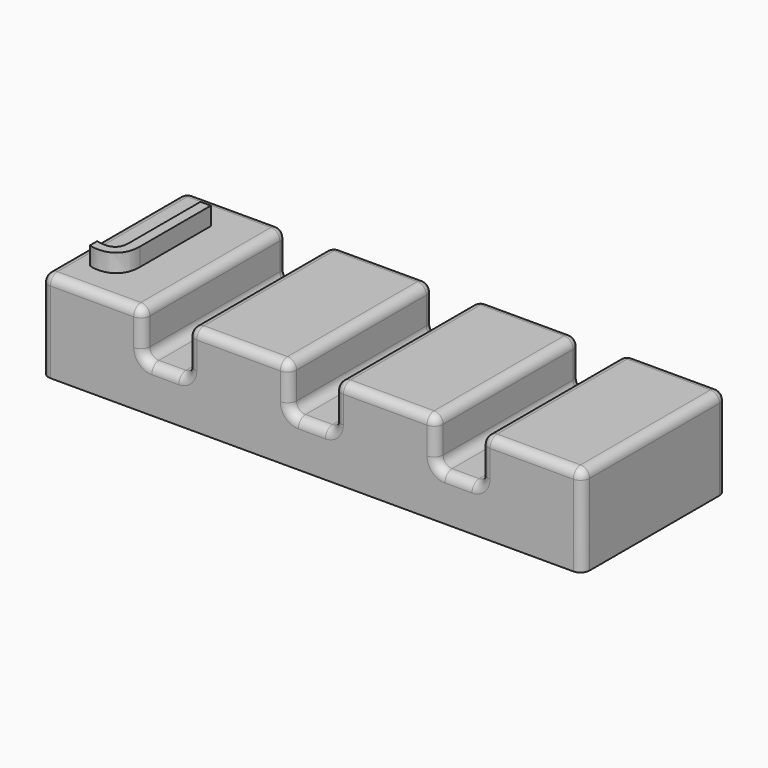
from build123d import *

# Parameters (mm, degrees)
F0_W         = 76.2
F0_H         = 25.4
F1_DEPTH     = 12.7
F2_W         = 6.35
F2_H         = 12.7
F3_DEPTH     = 25.401
F4_R         = 1.27
F5_T         = -2.54
F6_TEXT_SIZE = 17.6218719894
F7_DEPTH     = 2.54


# Not quite as in the source:
# - Text() gives the source's letters only with a copy of the font that has no kerning and outlines rounded to 1/6400 em; it was checked with that copy


with BuildPart() as f1:
    # F0 (on Top) → F1 (new body)
    with BuildSketch(Plane.XY):
        Rectangle(F0_W, F0_H)
    extrude(amount=F1_DEPTH)

    # F2 (on face) → F3 (cut, through all)
    with BuildSketch(Plane.XZ.offset(12.7)):
        with Locations((20.6502, 12.7)):
            Rectangle(F2_W, F2_H)
        with Locations((-20.6502, 12.7)):
            Rectangle(F2_W, F2_H)
        with Locations((0, 12.7)):
            Rectangle(F2_W, F2_H)
    extrude(amount=-F3_DEPTH, mode=Mode.SUBTRACT)

    # F4
    f4_edges = [f1.edges().sort_by_distance(p)[0] for p in [
        (-23.8252, 0, 12.7),
        (-30.9626, -12.7, 12.7),
        (-38.1, 0, 12.7),
        (-30.9626, 12.7, 12.7),
        (-3.175, 0, 12.7),
        (-10.3251, -12.7, 12.7),
        (-17.4752, 0, 12.7),
        (-10.3251, 12.7, 12.7),
        (17.4752, 0, 12.7),
        (10.3251, -12.7, 12.7),
        (3.175, 0, 12.7),
        (10.3251, 12.7, 12.7),
        (38.1, 0, 12.7),
        (30.9626, -12.7, 12.7),
        (23.8252, 0, 12.7),
        (30.9626, 12.7, 12.7),
        (-20.6502, -12.7, 6.35),
        (-17.4752, 0, 6.35),
        (-20.6502, 12.7, 6.35),
        (-23.8252, 0, 6.35),
        (0, -12.7, 6.35),
        (3.175, 0, 6.35),
        (0, 12.7, 6.35),
        (-3.175, 0, 6.35),
        (20.6502, -12.7, 6.35),
        (23.8252, 0, 6.35),
        (20.6502, 12.7, 6.35),
        (17.4752, 0, 6.35),
        (38.1, -12.7, 6.35),
        (38.1, 12.7, 6.35),
        (-38.1, -12.7, 6.35),
        (-38.1, 12.7, 6.35),
        (-23.8252, 12.7, 9.525),
        (-17.4752, 12.7, 9.525),
        (-3.175, 12.7, 9.525),
        (3.175, 12.7, 9.525),
        (17.4752, 12.7, 9.525),
        (23.8252, 12.7, 9.525),
        (-23.8252, -12.7, 9.525),
        (-17.4752, -12.7, 9.525),
        (-3.175, -12.7, 9.525),
        (3.175, -12.7, 9.525),
        (17.4752, -12.7, 9.525),
        (23.8252, -12.7, 9.525),
    ]]
    fillet(f4_edges, radius=F4_R)

    # F5
    f5_openings = [f1.faces().sort_by_distance(p)[0] for p in [
        (0, 0, 0),
    ]]
    offset(amount=F5_T, openings=f5_openings)

    # F6 (on face) → F7 (join)
    with BuildSketch(Plane.XY.offset(12.7)):
        with Locations((-33.5416737944, -5.0094374456)):
            Text('J', F6_TEXT_SIZE, font='Open Sans', text_align=(TextAlign.LEFT, TextAlign.BOTTOM))
    extrude(amount=F7_DEPTH)


solid = f1.part
